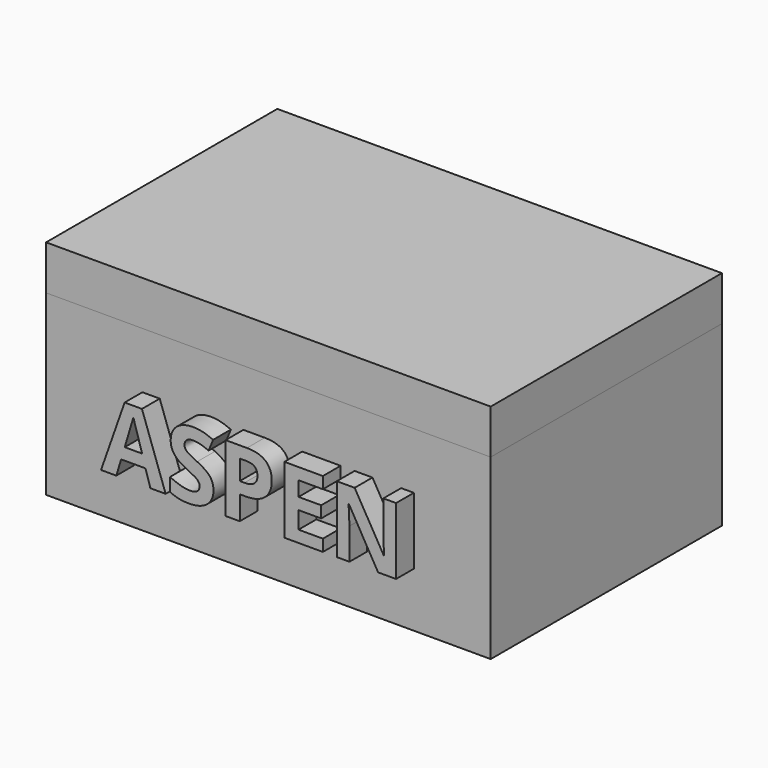
from build123d import *

# Parameters (mm, degrees)
F0_W         = 100
F0_H         = 65
F1_DEPTH     = 40
F2_T         = -2
F3_W         = 100
F3_H         = 65
F4_DEPTH     = 10
F5_T         = -3
F6_W         = 95.6
F6_H         = 60.6
F6_W_2       = 94
F6_H_2       = 59
F7_DEPTH     = 2
F9_TEXT_SIZE = 21.0526600332
F10_DEPTH    = 5


# Not quite as in the source:
# - Text() gives the source's letters only with a copy of the font that has no kerning and outlines rounded to 1/6400 em; it was checked with that copy


with BuildPart() as f1:
    # F0 (on Top) → F1 (new body)
    with BuildSketch(Plane.XY):
        with Locations((-25.6192844361, 16.6141179204)):
            Rectangle(F0_W, F0_H)
    extrude(amount=F1_DEPTH)

    # F2
    f2_openings = [f1.faces().sort_by_distance(p)[0] for p in [
        (-25.619284, 16.614118, 40),
    ]]
    offset(amount=F2_T, openings=f2_openings)

    # F9 (on face) → F10 (join)
    with BuildSketch(Plane.XZ.offset(15.8858820796)):
        with Locations((-59.2590132371, 12.2762772771)):
            Text('ASPEN', F9_TEXT_SIZE, font='Open Sans', font_style=FontStyle.BOLD, text_align=(TextAlign.LEFT, TextAlign.BOTTOM))
    extrude(amount=F10_DEPTH)


with BuildPart() as f4:
    # F3 (on face) → F4 (new body)
    with BuildSketch(Plane.XY.offset(40)):
        with Locations((-25.6192844361, 16.6141179204)):
            Rectangle(F3_W, F3_H)
    extrude(amount=F4_DEPTH)

    # F5
    f5_openings = [f4.faces().sort_by_distance(p)[0] for p in [
        (-25.619284, 16.614118, 40),
    ]]
    offset(amount=F5_T, openings=f5_openings)

    # F6 (on face) → F7 (join)
    with BuildSketch(Plane(origin=(0, 0, 40), x_dir=(1, 0, 0), z_dir=(0, 0, -1))):
        with Locations((-25.6192844361, -16.6141179204)):
            Rectangle(F6_W, F6_H)
        with Locations((-25.6192844361, -16.6141179204)):
            Rectangle(F6_W_2, F6_H_2, mode=Mode.SUBTRACT)
    extrude(amount=F7_DEPTH)


solid = Compound([f1.part, f4.part])
